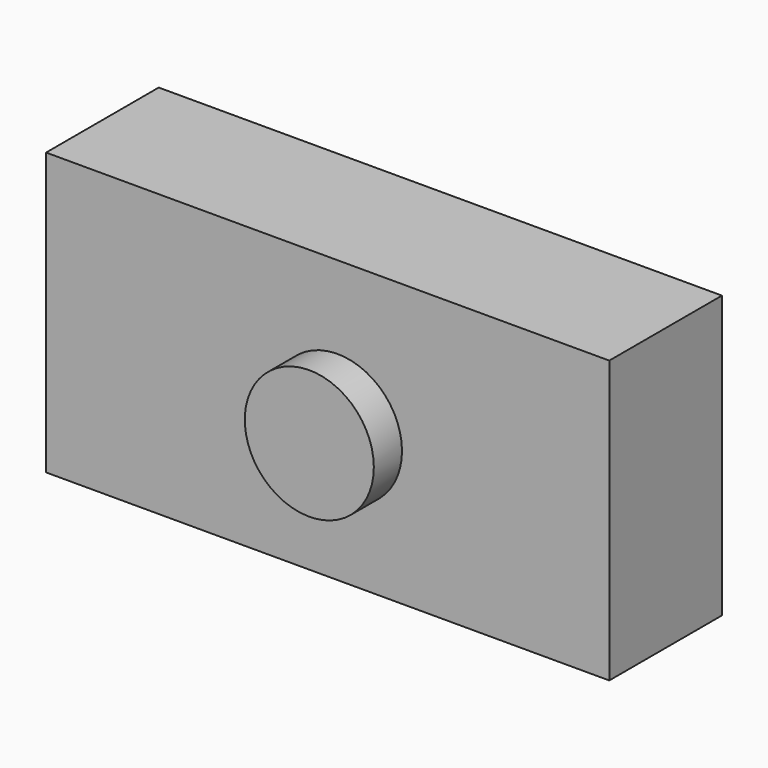
from build123d import *

# Parameters (mm, degrees)
F0_W     = 101.6
F0_H     = 50.8
F1_DEPTH = 25.4
F2_R     = 11.6399110946
F3_DEPTH = 6.35


# Not quite as in the source:
# - a feature of the source that left no trace in its solid (it failed there, or was rolled back) is left out


with BuildPart() as f1:
    # F0 (on Front) → F1 (new body)
    with BuildSketch(Plane.XZ):
        with Locations((-1.7657391727, 1.1206692427)):
            Rectangle(F0_W, F0_H)
    extrude(amount=F1_DEPTH)

    # F2 (on face) → F3 (join)
    with BuildSketch(Plane.XZ.offset(25.4)):
        Circle(F2_R)
    extrude(amount=F3_DEPTH)


solid = f1.part
